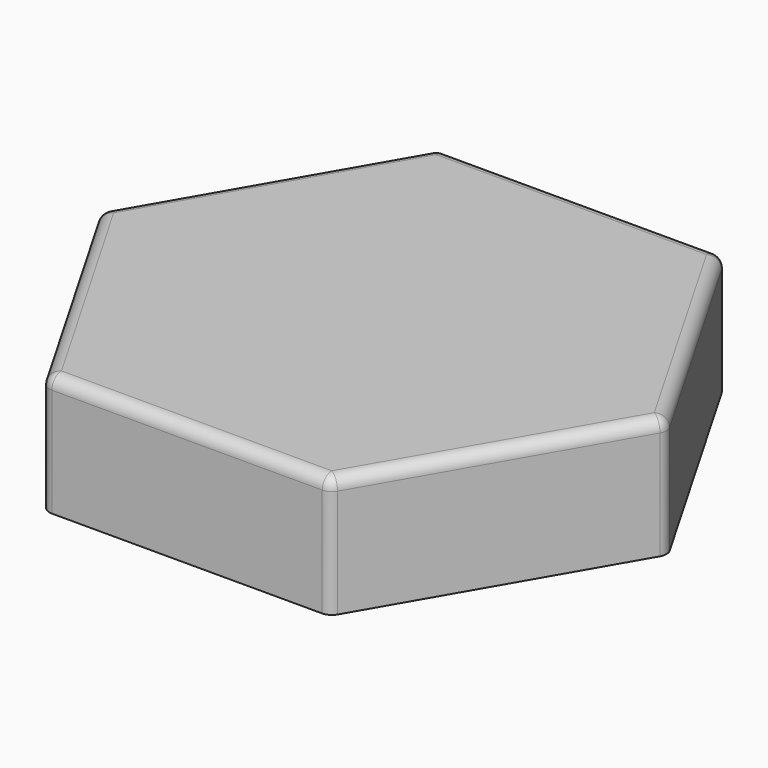
from build123d import *

# Parameters (mm, degrees)
F1_DEPTH = 3
F3_DEPTH = 10
F4_R     = 1
F5_DEPTH = 5


with BuildPart() as f1:
    # F0 (on Top) → F1 (new body)
    with BuildSketch(Plane.XY):
        Polygon((5.7735026919, 10), (-5.7735026919, 10), (-11.5470053838, 0), (-5.7735026919, -10), (5.7735026919, -10), (11.5470053838, 0), align=None)
        with BuildLine():
            ThreePointArc((-3.3867513459, 4.1339745962), (-3.3867513459, 5.8660254038), (-1.8867513459, 5))
            Line((-1.8867513459, 5), (1.8867513459, 5))
            ThreePointArc((1.8867513459, 5), (2.8867513459, 6), (3.8867513459, 5))
            ThreePointArc((3.8867513459, 5), (3.7527767497, 4.5), (3.3867513459, 4.1339745962))
            Line((3.3867513459, 4.1339745962), (5.2735026919, 0.8660254038))
            ThreePointArc((5.2735026919, 0.8660254038), (6.2735026919, 0.8660254038), (6.7735026919, 0))
            ThreePointArc((6.7735026919, 0), (6.2735026919, -0.8660254038), (5.2735026919, -0.8660254038))
            Line((5.2735026919, -0.8660254038), (3.3867513459, -4.1339745962))
            ThreePointArc((3.3867513459, -4.1339745962), (3.7527767497, -4.5), (3.8867513459, -5))
            ThreePointArc((3.8867513459, -5), (2.8867513459, -6), (1.8867513459, -5))
            Line((1.8867513459, -5), (-1.8867513459, -5))
            ThreePointArc((-1.8867513459, -5), (-3.3867513459, -5.8660254038), (-3.3867513459, -4.1339745962))
            Line((-3.3867513459, -4.1339745962), (-5.2735026919, -0.8660254038))
            ThreePointArc((-5.2735026919, -0.8660254038), (-6.7735026919, 0), (-5.2735026919, 0.8660254038))
            Line((-5.2735026919, 0.8660254038), (-3.3867513459, 4.1339745962))
        make_face(mode=Mode.SUBTRACT)
        with BuildLine():
            Line((1.8867513459, 5), (-1.8867513459, 5))
            ThreePointArc((-1.8867513459, 5), (-2.3867513459, 4.1339745962), (-3.3867513459, 4.1339745962))
            Line((-3.3867513459, 4.1339745962), (-5.2735026919, 0.8660254038))
            ThreePointArc((-5.2735026919, 0.8660254038), (-4.9074772881, 0.5), (-4.7735026919, 0))
            ThreePointArc((-4.7735026919, 0), (-4.9074772881, -0.5), (-5.2735026919, -0.8660254038))
            Line((-5.2735026919, -0.8660254038), (-3.3867513459, -4.1339745962))
            ThreePointArc((-3.3867513459, -4.1339745962), (-2.3867513459, -4.1339745962), (-1.8867513459, -5))
            Line((-1.8867513459, -5), (1.8867513459, -5))
            ThreePointArc((1.8867513459, -5), (2.3867513459, -4.1339745962), (3.3867513459, -4.1339745962))
            Line((3.3867513459, -4.1339745962), (5.2735026919, -0.8660254038))
            ThreePointArc((5.2735026919, -0.8660254038), (4.7735026919, 0), (5.2735026919, 0.8660254038))
            Line((5.2735026919, 0.8660254038), (3.3867513459, 4.1339745962))
            ThreePointArc((3.3867513459, 4.1339745962), (2.3867513459, 4.1339745962), (1.8867513459, 5))
        make_face()
    extrude(amount=F1_DEPTH)

    # F2 (on face) → F3 (join)
    with BuildSketch(Plane.XY.offset(3)):
        Polygon((11.7779454915, 20.4), (-11.7779454915, 20.4), (-23.5558909829, 0), (-11.7779454915, -20.4), (11.7779454915, -20.4), (23.5558909829, 0), align=None)
        Polygon((5.7735026919, 10), (11.5470053838, 0), (5.7735026919, -10), (-5.7735026919, -10), (-11.5470053838, 0), (-5.7735026919, 10), align=None, mode=Mode.SUBTRACT)
        Polygon((11.7779454915, 20.4), (-11.7779454915, 20.4), (-23.5558909829, 0), (-11.7779454915, -20.4), (11.7779454915, -20.4), (23.5558909829, 0), align=None)
    extrude(amount=F3_DEPTH)

    # F4
    f4_edges = [f1.edges().sort_by_distance(p)[0] for p in [
        (-17.666918, 10.2, 13),
        (-17.666918, -10.2, 13),
        (0, -20.4, 13),
        (17.666918, -10.2, 13),
        (17.666918, 10.2, 13),
        (0, 20.4, 13),
        (-11.777945, 20.4, 8),
        (11.777945, 20.4, 8),
        (23.555891, 0, 8),
        (-23.555891, 0, 8),
        (11.777945, -20.4, 8),
        (-11.777945, -20.4, 8),
    ]]
    fillet(f4_edges, radius=F4_R)

    # F5 (cut): faces of the model
    f5_faces = [f1.faces().sort_by_distance(p)[0] for p in [
        (-2.8867513459, -5, 3),
        (2.8867513459, -5, 3),
        (5.7735026919, 0, 3),
        (2.8867513459, 5, 3),
        (-2.8867513459, 5, 3),
        (-5.7735026919, 0, 3),
    ]]
    extrude(f5_faces, amount=-F5_DEPTH, mode=Mode.SUBTRACT)


solid = f1.part
